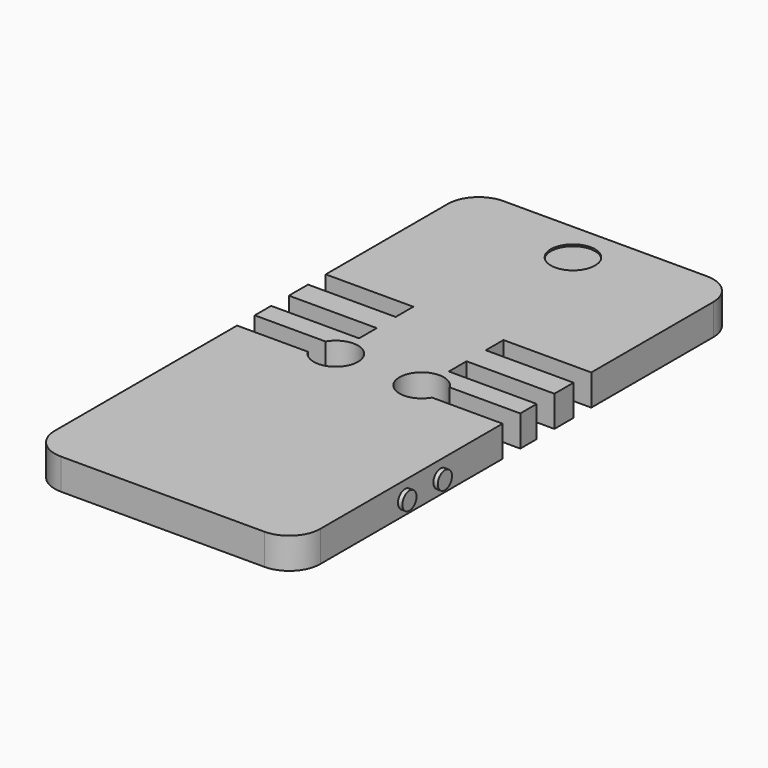
from build123d import *

# Parameters (mm, degrees)
F0_W      = 60
F0_H      = 125
F1_DEPTH  = 7
F2_R      = 7
F3_R      = 7
F4_R      = 7
F5_R      = 2
F6_DEPTH  = 1
F9_W      = 20
F9_H      = 5
F10_DEPTH = 88.1
F7_R      = 5
F12_DEPTH = 0.4


# Not quite as in the source:
# - the program builds the solid bodies; features that only make, move or delete a surface that nothing else refers to are left out


with BuildPart() as f1:
    # F0 (on Top) → F1 (new body)
    with BuildSketch(Plane.XY):
        with Locations((4.798640497, -0.129804003)):
            Rectangle(F0_W, F0_H)
    extrude(amount=F1_DEPTH)

    # F2
    f2_edges = [f1.edges().sort_by_distance(p)[0] for p in [
        (-25.20136, -62.629804, 3.5),
    ]]
    fillet(f2_edges, radius=F2_R)

    # F3
    f3_edges = [f1.edges().sort_by_distance(p)[0] for p in [
        (-25.20136, 62.370196, 3.5),
        (34.79864, -62.629804, 3.5),
    ]]
    fillet(f3_edges, radius=F3_R)

    # F4
    f4_edges = [f1.edges().sort_by_distance(p)[0] for p in [
        (34.79864, 62.370196, 3.5),
    ]]
    fillet(f4_edges, radius=F4_R)

    # F5 (on face) → F6 (join)
    with BuildSketch(Plane.YZ.offset(34.798640497)):
        with Locations((-31.6818073764, 3.2178394031)):
            Circle(F5_R)
        with Locations((-21.6818073764, 3.2178394031)):
            Circle(F5_R)
    extrude(amount=F6_DEPTH)

    # F9 (on Top) → F10 (cut)
    with BuildSketch(Plane.XY):
        with Locations((-15.4034045642, 18.4103432111)):
            Rectangle(F9_W, F9_H)
        with Locations((24.9580888633, 18.4103432111)):
            Rectangle(F9_W, F9_H)
        with Locations((-15.3402814512, 8.0003063194)):
            Rectangle(F9_W, F9_H)
        with Locations((24.940414155, 8.0003063194)):
            Rectangle(F9_W, F9_H)
        with BuildLine():
            Line((-9.2095649145, 0.8613835648), (-25.9844651689, 0.8613835648))
            Line((-25.9844651689, 0.8613835648), (-25.9844651689, -4.1386164352))
            Line((-25.9844651689, -4.1386164352), (-9.2095649145, -4.1386164352))
            ThreePointArc((-9.2095649145, -4.1386164352), (-9.8794378956, -1.6386164352), (-9.2095649145, 0.8613835648))
        make_face()
        with BuildLine():
            ThreePointArc((0.1205621044, -1.6386164352), (-3.5853426701, 3.1910126962), (-9.2095649145, 0.8613835648))
            ThreePointArc((-9.2095649145, 0.8613835648), (-9.8794378956, -1.6386164352), (-9.2095649145, -4.1386164352))
            ThreePointArc((-9.2095649145, -4.1386164352), (-3.5853426701, -6.4682455667), (0.1205621044, -1.6386164352))
        make_face()
        with BuildLine():
            Line((36.6257494559, -4.1386164352), (36.6257494559, 0.8613835648))
            Line((36.6257494559, 0.8613835648), (18.8484872035, 0.8613835648))
            ThreePointArc((18.8484872035, 0.8613835648), (9.5183601846, -1.6386164352), (18.8484872035, -4.1386164352))
            Line((18.8484872035, -4.1386164352), (36.6257494559, -4.1386164352))
        make_face()
    extrude(amount=F10_DEPTH, mode=Mode.SUBTRACT)

    # F7 (on face) → F12 (cut)
    with BuildSketch(Plane.XY.offset(7)):
        with Locations((4.798640497, 53.2364137471)):
            Circle(F7_R)
    extrude(amount=-F12_DEPTH, mode=Mode.SUBTRACT)


solid = f1.part
